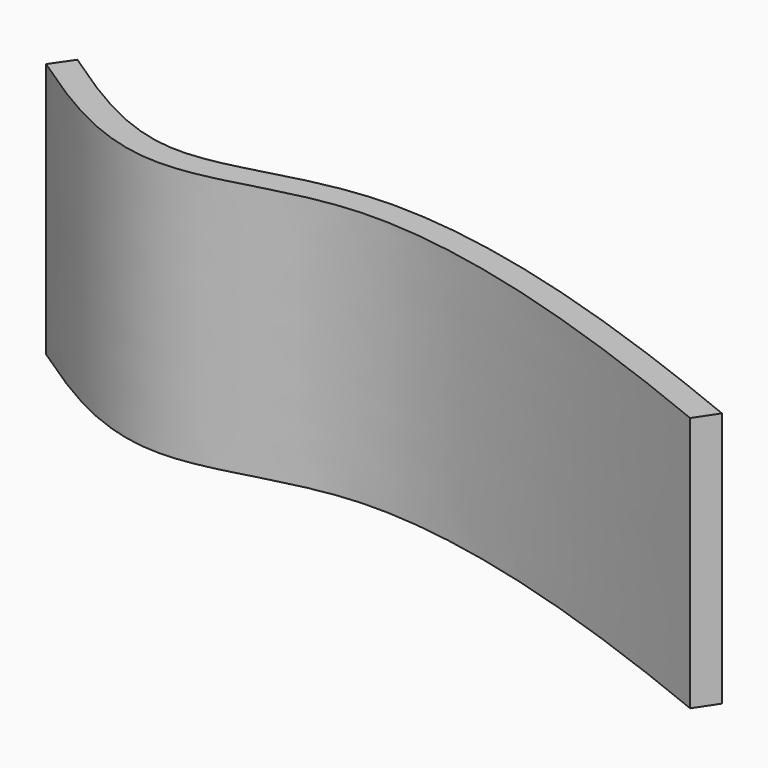
from build123d import *

# Parameters (mm, degrees)
F1_DEPTH = 25.4


# Not quite as in the source:
# - the dataset's text gives a spline's control points without its knots; the knots are read off the source's solid


with BuildPart() as f1:
    # F0 (on Top) → F1 (new body)
    with BuildSketch(Plane.XY):
        with BuildLine():
            add(Edge.make_bspline(
                [(0, 0), (4.8630121686, -3.3181693183), (15.2759533832, -10.2863001285), (33.6045572417, 0.6674747862), (61.3874158585, -9.0882847366), (76.2, -15.1677737013)],
                knots=[0, 0, 0, 0, 0.2707501019, 0.5540723526, 1, 1, 1, 1], degree=3))
            Line((0, 0), (-1.4316056384, -2.0981194666))
            add(Edge.make_bspline(
                [(-1.4316056384, -2.0981194666), (-0.305996139, -2.8661543338), (1.9998032211, -4.4327197905), (5.0097253075, -6.268006745), (7.5045686592, -7.5391109076), (9.4249187415, -8.3600980332), (11.4008720789, -9.011643965), (13.0977492135, -9.3772229214), (14.4850786594, -9.5391270908), (15.8873355108, -9.6028096872), (17.5881476385, -9.5063110655), (19.5630706723, -9.1910859259), (21.4888236888, -8.7465684012), (23.3941142493, -8.2329342762), (25.3061689722, -7.7015241141), (27.2506768842, -7.1981544829), (29.2521403856, -6.7649140684), (30.9883432325, -6.495671256), (32.432175868, -6.3548203249), (33.9170805519, -6.271245784), (35.8974527802, -6.2764985504), (39.2909372261, -6.5095961507), (43.9050753216, -7.2012689856), (49.8757255396, -8.581455062), (56.1339830831, -10.4094320792), (62.5415228715, -12.5792199237), (68.8039749461, -14.9230291487), (72.8551010948, -16.5436750777), (74.7683943279, -17.3261530312)],
                knots=[0, 0, 0, 0, 0.0625, 0.125, 0.15625, 0.1875, 0.21875, 0.25, 0.265625, 0.28125, 0.3125, 0.34375, 0.375, 0.40625, 0.4375, 0.46875, 0.5, 0.53125, 0.546875, 0.5625, 0.59375, 0.625, 0.6875, 0.75, 0.8125, 0.875, 0.9375, 0.9952895991, 0.9952895991, 0.9952895991, 0.9952895991], degree=3))
            Line((74.7683943616, -17.3261529488), (76.2, -15.1677737013))
        make_face()
    extrude(amount=F1_DEPTH)


solid = f1.part
